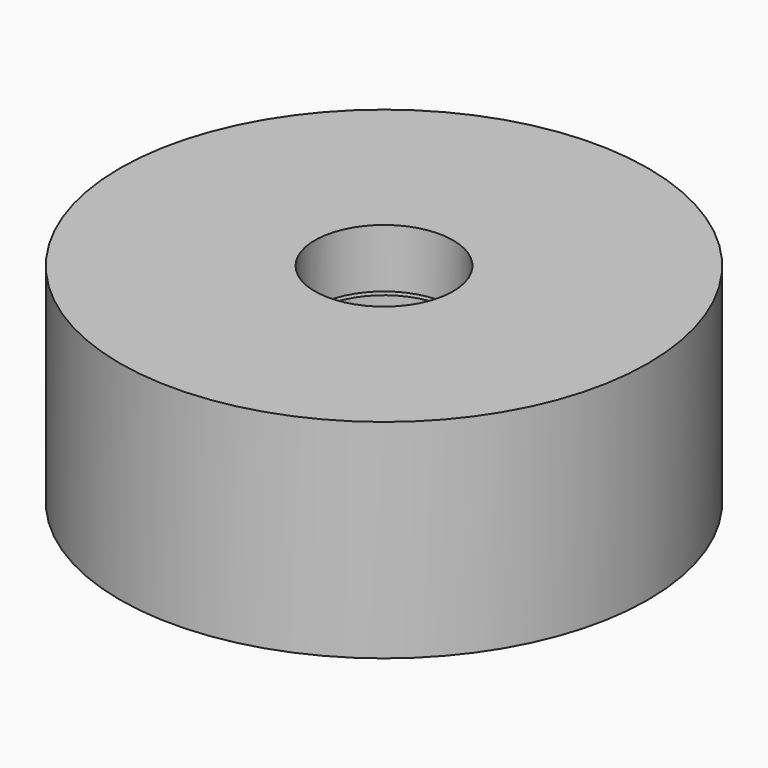
from build123d import *

# Parameters (mm, degrees)
F0_R            = 12.7
F0_R_2          = 4.5
F1_DEPTH        = 9.525
F2_R            = 2.54
F6_COPIES_COUNT = 10
F9_COUNT        = 15
F9_ANGLE        = 336


# Not quite as in the source:
# - a feature of the source that left no trace in its solid (it failed there, or was rolled back) is left out
# - a pattern or mirror of a feature is missing from the dataset's text; its kind, count and spacing are read off the source's solid


with BuildPart() as f1:
    # F0 (on Top) → F1 (new body)
    with BuildSketch(Plane.XY):
        Circle(F0_R)
        Circle(F0_R_2, mode=Mode.SUBTRACT)
    extrude(amount=F1_DEPTH)

    # F2 (on Front) → F3 (revolve, cut)
    with BuildSketch(Plane.XZ):
        with Locations((7.5, 9.8171)):
            Circle(F2_R)
        with BuildLine():
            ThreePointArc((5.2521, 9.8171), (7.5, 12.065), (9.7479, 9.8171))
            ThreePointArc((9.7479, 9.8171), (7.5, 7.5692), (5.2521, 9.8171))
        make_face(mode=Mode.SUBTRACT)
        with Locations((12.7, 5.08)):
            Circle(F2_R)
        with BuildLine():
            ThreePointArc((12.7, 7.33679), (14.2957915127, 6.6757915127), (14.95679, 5.08))
            ThreePointArc((14.95679, 5.08), (14.2957915127, 3.4842084873), (12.7, 2.82321))
            ThreePointArc((12.7, 2.82321), (10.44321, 5.08), (12.7, 7.33679))
        make_face(mode=Mode.SUBTRACT)
        with BuildLine():
            Line((12.7, 2.82321), (12.7, 7.33679))
            ThreePointArc((12.7, 7.33679), (10.44321, 5.08), (12.7, 2.82321))
        make_face()
        with BuildLine():
            ThreePointArc((12.7, 2.82321), (14.2957915127, 3.4842084873), (14.95679, 5.08))
            ThreePointArc((14.95679, 5.08), (14.2957915127, 6.6757915127), (12.7, 7.33679))
            Line((12.7, 7.33679), (12.7, 2.82321))
        make_face()
        with BuildLine():
            Line((5.2521, 9.8171), (9.7479, 9.8171))
            ThreePointArc((9.7479, 9.8171), (7.5, 12.065), (5.2521, 9.8171))
        make_face()
        with BuildLine():
            ThreePointArc((5.2521, 9.8171), (7.5, 7.5692), (9.7479, 9.8171))
            Line((9.7479, 9.8171), (5.2521, 9.8171))
        make_face()
    revolve(axis=Axis((0, 0, 9.525), (0, 0, 1)), mode=Mode.SUBTRACT)


with BuildPart() as f5:
    # F4 (on Front) → F5 (revolve)
    with BuildSketch(Plane.XZ):
        with BuildLine():
            ThreePointArc((13.0270650942, 7.5988545858), (14.608185701, 6.7564329185), (15.24, 5.08))
            ThreePointArc((15.24, 5.08), (14.9954010018, 3.9924641427), (14.3087131961, 3.1143851209))
            Line((14.3087131961, 3.1143851209), (14.9143021554, 0))
            Line((14.9143021554, 0), (17.2, 0))
            Line((17.2, 0), (17.2, 13.5538493477))
            Line((17.2, 13.5538493477), (4.5, 13.5538493477))
            Line((4.5, 13.5538493477), (4.5, 9.7438493477))
            Line((4.5, 9.7438493477), (4.9610564516, 9.7438493477))
            ThreePointArc((4.9610564516, 9.7438493477), (7.4633708649, 12.3568358734), (10.04, 9.8171))
            ThreePointArc((10.04, 9.8171), (10.0399734216, 9.8054802973), (10.039893687, 9.7938608378))
            Line((10.039893687, 9.7938608378), (13.0270650942, 9.7938608378))
            Line((13.0270650942, 9.7938608378), (13.0270650942, 7.5988545858))
        make_face()
    revolve(axis=Axis((0, 0, 9.525), (0, 0, 1)))


with BuildPart() as f6:
    # F2 (on Front) → F6 (revolve)
    with BuildSketch(Plane.XZ):
        with BuildLine():
            Line((5.2521, 9.8171), (9.7479, 9.8171))
            ThreePointArc((9.7479, 9.8171), (7.5, 12.065), (5.2521, 9.8171))
        make_face()
    revolve(axis=Axis((7.5, 0, 9.8171), (1, 0, 0)))


with BuildPart() as f6_copies_1:
    # F6_copies: instance of F6
    add(f6.part.rotate(Axis((0, 0, 0), (0, 0, 1)), 1 * 360 / F6_COPIES_COUNT))


with BuildPart() as f6_copies_2:
    # F6_copies: instance of F6
    add(f6.part.rotate(Axis((0, 0, 0), (0, 0, 1)), 2 * 360 / F6_COPIES_COUNT))


with BuildPart() as f6_copies_3:
    # F6_copies: instance of F6
    add(f6.part.rotate(Axis((0, 0, 0), (0, 0, 1)), 3 * 360 / F6_COPIES_COUNT))


with BuildPart() as f6_copies_4:
    # F6_copies: instance of F6
    add(f6.part.rotate(Axis((0, 0, 0), (0, 0, 1)), 4 * 360 / F6_COPIES_COUNT))


with BuildPart() as f6_copies_5:
    # F6_copies: instance of F6
    add(f6.part.rotate(Axis((0, 0, 0), (0, 0, 1)), 5 * 360 / F6_COPIES_COUNT))


with BuildPart() as f6_copies_6:
    # F6_copies: instance of F6
    add(f6.part.rotate(Axis((0, 0, 0), (0, 0, 1)), 6 * 360 / F6_COPIES_COUNT))


with BuildPart() as f6_copies_7:
    # F6_copies: instance of F6
    add(f6.part.rotate(Axis((0, 0, 0), (0, 0, 1)), 7 * 360 / F6_COPIES_COUNT))


with BuildPart() as f6_copies_8:
    # F6_copies: instance of F6
    add(f6.part.rotate(Axis((0, 0, 0), (0, 0, 1)), 8 * 360 / F6_COPIES_COUNT))


with BuildPart() as f6_copies_9:
    # F6_copies: instance of F6
    add(f6.part.rotate(Axis((0, 0, 0), (0, 0, 1)), 9 * 360 / F6_COPIES_COUNT))


with BuildPart() as f7:
    # F2 (on Front) → F7 (revolve)
    with BuildSketch(Plane.XZ):
        with BuildLine():
            ThreePointArc((12.7, 2.82321), (14.2957915127, 3.4842084873), (14.95679, 5.08))
            ThreePointArc((14.95679, 5.08), (14.2957915127, 6.6757915127), (12.7, 7.33679))
            Line((12.7, 7.33679), (12.7, 2.82321))
        make_face()
    revolve(axis=Axis((12.7, 0, 5.08), (0, 0, -1)))


with BuildPart() as f9_1:
    # F9: instance of F7
    add(f7.part.rotate(Axis((0, 0, 9.525), (0, 0, 1)), 1 * F9_ANGLE / (F9_COUNT - 1)))


with BuildPart() as f9_2:
    # F9: instance of F7
    add(f7.part.rotate(Axis((0, 0, 9.525), (0, 0, 1)), 2 * F9_ANGLE / (F9_COUNT - 1)))


with BuildPart() as f9_3:
    # F9: instance of F7
    add(f7.part.rotate(Axis((0, 0, 9.525), (0, 0, 1)), 3 * F9_ANGLE / (F9_COUNT - 1)))


with BuildPart() as f9_4:
    # F9: instance of F7
    add(f7.part.rotate(Axis((0, 0, 9.525), (0, 0, 1)), 4 * F9_ANGLE / (F9_COUNT - 1)))


with BuildPart() as f9_5:
    # F9: instance of F7
    add(f7.part.rotate(Axis((0, 0, 9.525), (0, 0, 1)), 5 * F9_ANGLE / (F9_COUNT - 1)))


with BuildPart() as f9_6:
    # F9: instance of F7
    add(f7.part.rotate(Axis((0, 0, 9.525), (0, 0, 1)), 6 * F9_ANGLE / (F9_COUNT - 1)))


with BuildPart() as f9_7:
    # F9: instance of F7
    add(f7.part.rotate(Axis((0, 0, 9.525), (0, 0, 1)), 7 * F9_ANGLE / (F9_COUNT - 1)))


with BuildPart() as f9_8:
    # F9: instance of F7
    add(f7.part.rotate(Axis((0, 0, 9.525), (0, 0, 1)), 8 * F9_ANGLE / (F9_COUNT - 1)))


with BuildPart() as f9_9:
    # F9: instance of F7
    add(f7.part.rotate(Axis((0, 0, 9.525), (0, 0, 1)), 9 * F9_ANGLE / (F9_COUNT - 1)))


with BuildPart() as f9_10:
    # F9: instance of F7
    add(f7.part.rotate(Axis((0, 0, 9.525), (0, 0, 1)), 10 * F9_ANGLE / (F9_COUNT - 1)))


with BuildPart() as f9_11:
    # F9: instance of F7
    add(f7.part.rotate(Axis((0, 0, 9.525), (0, 0, 1)), 11 * F9_ANGLE / (F9_COUNT - 1)))


with BuildPart() as f9_12:
    # F9: instance of F7
    add(f7.part.rotate(Axis((0, 0, 9.525), (0, 0, 1)), 12 * F9_ANGLE / (F9_COUNT - 1)))


with BuildPart() as f9_13:
    # F9: instance of F7
    add(f7.part.rotate(Axis((0, 0, 9.525), (0, 0, 1)), 13 * F9_ANGLE / (F9_COUNT - 1)))


with BuildPart() as f9_14:
    # F9: instance of F7
    add(f7.part.rotate(Axis((0, 0, 9.525), (0, 0, 1)), 14 * F9_ANGLE / (F9_COUNT - 1)))


solid = Compound([f1.part, f5.part, f6.part, f6_copies_1.part, f6_copies_2.part, f6_copies_3.part, f6_copies_4.part, f6_copies_5.part, f6_copies_6.part, f6_copies_7.part, f6_copies_8.part, f6_copies_9.part, f7.part, f9_1.part, f9_2.part, f9_3.part, f9_4.part, f9_5.part, f9_6.part, f9_7.part, f9_8.part, f9_9.part, f9_10.part, f9_11.part, f9_12.part, f9_13.part, f9_14.part])
